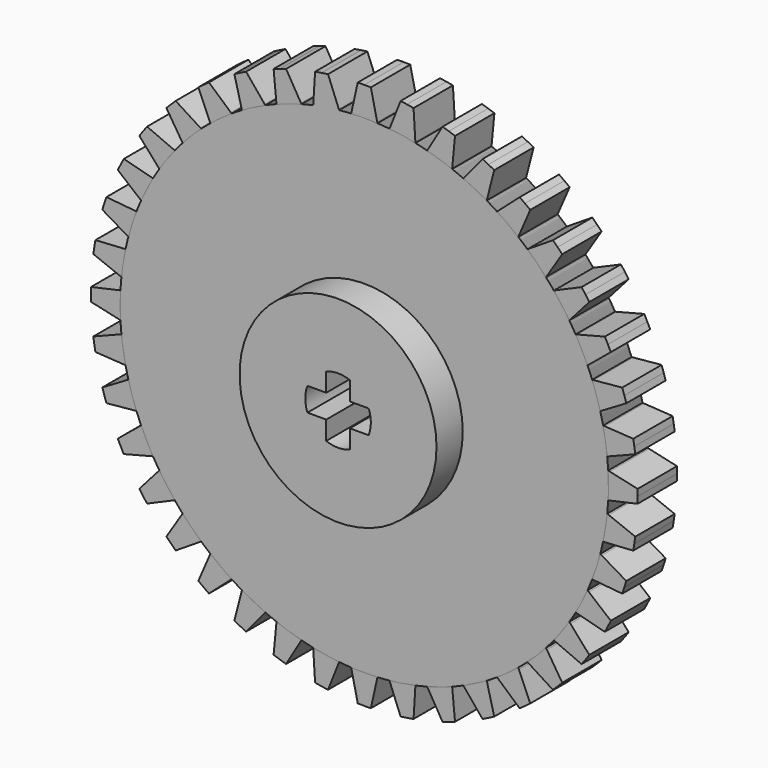
from build123d import *

# Parameters (mm, degrees)
F0_R     = 7.5
F1_DEPTH = 1.875
F3_COUNT = 40
F4_DEPTH = 4.375
F6_DEPTH = 25


with BuildPart() as f1:
    # F0 (on Front) → F1 (new body, symmetric)
    with BuildSketch(Plane.XZ):
        with BuildLine():
            Line((0.7872608089, 3.3734422161), (0.3026279116, 5.5503142364))
            Line((0.3026279116, 5.5503142364), (-0.1973720884, 5.5563175026))
            ThreePointArc((-0.1973720884, 5.5563175026), (-0.4473901074, 5.554816632), (-0.6973720884, 5.5503142364))
            Line((-0.6973720884, 5.5503142364), (-1.1705333394, 3.424970509))
            Line((-1.1705333394, 3.424970509), (-1.1973720884, 3.3044163286))
            ThreePointArc((-1.1973720884, 3.3044163286), (-0.1973720884, 3.3313175026), (0.8026279116, 3.3044163286))
            Line((0.8026279116, 3.3044163286), (0.7872608089, 3.3734422161))
        make_face()
        with BuildLine():
            ThreePointArc((18.4026279116, -15.2686824974), (13.303738977, -2.474934024), (0.8026279116, 3.3044163286))
            ThreePointArc((0.8026279116, 3.3044163286), (-0.1973720884, 3.3313175026), (-1.1973720884, 3.3044163286))
            ThreePointArc((-1.1973720884, 3.3044163286), (-12.9911205618, -28.7697935627), (18.4026279116, -15.2686824974))
        make_face()
        with Locations((-0.1973720884, -15.2686824974)):
            Circle(F0_R, mode=Mode.SUBTRACT)
    extrude(amount=F1_DEPTH, both=True)


with BuildPart() as f3_1:
    # F3: instance of F1
    add(f1.part.rotate(Axis((-0.1973720884, 1.875, -15.2686824974), (0, 1, 0)), 1 * 360 / F3_COUNT))


with BuildPart() as f3_2:
    # F3: instance of F1
    add(f1.part.rotate(Axis((-0.1973720884, 1.875, -15.2686824974), (0, 1, 0)), 2 * 360 / F3_COUNT))


with BuildPart() as f3_3:
    # F3: instance of F1
    add(f1.part.rotate(Axis((-0.1973720884, 1.875, -15.2686824974), (0, 1, 0)), 3 * 360 / F3_COUNT))


with BuildPart() as f3_4:
    # F3: instance of F1
    add(f1.part.rotate(Axis((-0.1973720884, 1.875, -15.2686824974), (0, 1, 0)), 4 * 360 / F3_COUNT))


with BuildPart() as f3_5:
    # F3: instance of F1
    add(f1.part.rotate(Axis((-0.1973720884, 1.875, -15.2686824974), (0, 1, 0)), 5 * 360 / F3_COUNT))


with BuildPart() as f3_6:
    # F3: instance of F1
    add(f1.part.rotate(Axis((-0.1973720884, 1.875, -15.2686824974), (0, 1, 0)), 6 * 360 / F3_COUNT))


with BuildPart() as f3_7:
    # F3: instance of F1
    add(f1.part.rotate(Axis((-0.1973720884, 1.875, -15.2686824974), (0, 1, 0)), 7 * 360 / F3_COUNT))


with BuildPart() as f3_8:
    # F3: instance of F1
    add(f1.part.rotate(Axis((-0.1973720884, 1.875, -15.2686824974), (0, 1, 0)), 8 * 360 / F3_COUNT))


with BuildPart() as f3_9:
    # F3: instance of F1
    add(f1.part.rotate(Axis((-0.1973720884, 1.875, -15.2686824974), (0, 1, 0)), 9 * 360 / F3_COUNT))


with BuildPart() as f3_10:
    # F3: instance of F1
    add(f1.part.rotate(Axis((-0.1973720884, 1.875, -15.2686824974), (0, 1, 0)), 10 * 360 / F3_COUNT))


with BuildPart() as f3_11:
    # F3: instance of F1
    add(f1.part.rotate(Axis((-0.1973720884, 1.875, -15.2686824974), (0, 1, 0)), 11 * 360 / F3_COUNT))


with BuildPart() as f3_12:
    # F3: instance of F1
    add(f1.part.rotate(Axis((-0.1973720884, 1.875, -15.2686824974), (0, 1, 0)), 12 * 360 / F3_COUNT))


with BuildPart() as f3_13:
    # F3: instance of F1
    add(f1.part.rotate(Axis((-0.1973720884, 1.875, -15.2686824974), (0, 1, 0)), 13 * 360 / F3_COUNT))


with BuildPart() as f3_14:
    # F3: instance of F1
    add(f1.part.rotate(Axis((-0.1973720884, 1.875, -15.2686824974), (0, 1, 0)), 14 * 360 / F3_COUNT))


with BuildPart() as f3_15:
    # F3: instance of F1
    add(f1.part.rotate(Axis((-0.1973720884, 1.875, -15.2686824974), (0, 1, 0)), 15 * 360 / F3_COUNT))


with BuildPart() as f3_16:
    # F3: instance of F1
    add(f1.part.rotate(Axis((-0.1973720884, 1.875, -15.2686824974), (0, 1, 0)), 16 * 360 / F3_COUNT))


with BuildPart() as f3_17:
    # F3: instance of F1
    add(f1.part.rotate(Axis((-0.1973720884, 1.875, -15.2686824974), (0, 1, 0)), 17 * 360 / F3_COUNT))


with BuildPart() as f3_18:
    # F3: instance of F1
    add(f1.part.rotate(Axis((-0.1973720884, 1.875, -15.2686824974), (0, 1, 0)), 18 * 360 / F3_COUNT))


with BuildPart() as f3_19:
    # F3: instance of F1
    add(f1.part.rotate(Axis((-0.1973720884, 1.875, -15.2686824974), (0, 1, 0)), 19 * 360 / F3_COUNT))


with BuildPart() as f3_20:
    # F3: instance of F1
    add(f1.part.rotate(Axis((-0.1973720884, 1.875, -15.2686824974), (0, 1, 0)), 20 * 360 / F3_COUNT))


with BuildPart() as f3_21:
    # F3: instance of F1
    add(f1.part.rotate(Axis((-0.1973720884, 1.875, -15.2686824974), (0, 1, 0)), 21 * 360 / F3_COUNT))


with BuildPart() as f3_22:
    # F3: instance of F1
    add(f1.part.rotate(Axis((-0.1973720884, 1.875, -15.2686824974), (0, 1, 0)), 22 * 360 / F3_COUNT))


with BuildPart() as f3_23:
    # F3: instance of F1
    add(f1.part.rotate(Axis((-0.1973720884, 1.875, -15.2686824974), (0, 1, 0)), 23 * 360 / F3_COUNT))


with BuildPart() as f3_24:
    # F3: instance of F1
    add(f1.part.rotate(Axis((-0.1973720884, 1.875, -15.2686824974), (0, 1, 0)), 24 * 360 / F3_COUNT))


with BuildPart() as f3_25:
    # F3: instance of F1
    add(f1.part.rotate(Axis((-0.1973720884, 1.875, -15.2686824974), (0, 1, 0)), 25 * 360 / F3_COUNT))


with BuildPart() as f3_26:
    # F3: instance of F1
    add(f1.part.rotate(Axis((-0.1973720884, 1.875, -15.2686824974), (0, 1, 0)), 26 * 360 / F3_COUNT))


with BuildPart() as f3_27:
    # F3: instance of F1
    add(f1.part.rotate(Axis((-0.1973720884, 1.875, -15.2686824974), (0, 1, 0)), 27 * 360 / F3_COUNT))


with BuildPart() as f3_28:
    # F3: instance of F1
    add(f1.part.rotate(Axis((-0.1973720884, 1.875, -15.2686824974), (0, 1, 0)), 28 * 360 / F3_COUNT))


with BuildPart() as f3_29:
    # F3: instance of F1
    add(f1.part.rotate(Axis((-0.1973720884, 1.875, -15.2686824974), (0, 1, 0)), 29 * 360 / F3_COUNT))


with BuildPart() as f3_30:
    # F3: instance of F1
    add(f1.part.rotate(Axis((-0.1973720884, 1.875, -15.2686824974), (0, 1, 0)), 30 * 360 / F3_COUNT))


with BuildPart() as f3_31:
    # F3: instance of F1
    add(f1.part.rotate(Axis((-0.1973720884, 1.875, -15.2686824974), (0, 1, 0)), 31 * 360 / F3_COUNT))


with BuildPart() as f3_32:
    # F3: instance of F1
    add(f1.part.rotate(Axis((-0.1973720884, 1.875, -15.2686824974), (0, 1, 0)), 32 * 360 / F3_COUNT))


with BuildPart() as f3_33:
    # F3: instance of F1
    add(f1.part.rotate(Axis((-0.1973720884, 1.875, -15.2686824974), (0, 1, 0)), 33 * 360 / F3_COUNT))


with BuildPart() as f3_34:
    # F3: instance of F1
    add(f1.part.rotate(Axis((-0.1973720884, 1.875, -15.2686824974), (0, 1, 0)), 34 * 360 / F3_COUNT))


with BuildPart() as f3_35:
    # F3: instance of F1
    add(f1.part.rotate(Axis((-0.1973720884, 1.875, -15.2686824974), (0, 1, 0)), 35 * 360 / F3_COUNT))


with BuildPart() as f3_36:
    # F3: instance of F1
    add(f1.part.rotate(Axis((-0.1973720884, 1.875, -15.2686824974), (0, 1, 0)), 36 * 360 / F3_COUNT))


with BuildPart() as f3_37:
    # F3: instance of F1
    add(f1.part.rotate(Axis((-0.1973720884, 1.875, -15.2686824974), (0, 1, 0)), 37 * 360 / F3_COUNT))


with BuildPart() as f3_38:
    # F3: instance of F1
    add(f1.part.rotate(Axis((-0.1973720884, 1.875, -15.2686824974), (0, 1, 0)), 38 * 360 / F3_COUNT))


with BuildPart() as f3_39:
    # F3: instance of F1
    add(f1.part.rotate(Axis((-0.1973720884, 1.875, -15.2686824974), (0, 1, 0)), 39 * 360 / F3_COUNT))


with BuildPart() as f4:
    # F0 (on Front) → F4 (new body, symmetric)
    with BuildSketch(Plane.XZ):
        with Locations((-0.1973720884, -15.2686824974)):
            Circle(F0_R)
    extrude(amount=F4_DEPTH, both=True)

    # F5 (on face) → F6 (cut)
    with BuildSketch(Plane.XZ.offset(4.375)):
        with BuildLine():
            ThreePointArc((2.1339367714, -16.1686824974), (2.2593474561, -15.7264270545), (2.3016279116, -15.2686824974))
            ThreePointArc((2.3016279116, -15.2686824974), (2.2593474561, -14.8109379402), (2.1339367714, -14.3686824974))
            Line((2.1339367714, -14.3686824974), (0.7026279116, -14.3686824974))
            Line((0.7026279116, -14.3686824974), (0.7026279116, -12.9373736375))
            ThreePointArc((0.7026279116, -12.9373736375), (-0.1973720884, -12.7696824974), (-1.0973720884, -12.9373736375))
            Line((-1.0973720884, -12.9373736375), (-1.0973720884, -14.3686824974))
            Line((-1.0973720884, -14.3686824974), (-2.5286809483, -14.3686824974))
            ThreePointArc((-2.5286809483, -14.3686824974), (-2.6963720884, -15.2686824974), (-2.5286809483, -16.1686824974))
            Line((-2.5286809483, -16.1686824974), (-1.0973720884, -16.1686824974))
            Line((-1.0973720884, -16.1686824974), (-1.0973720884, -17.5999913572))
            ThreePointArc((-1.0973720884, -17.5999913572), (-0.1973720884, -17.7676824974), (0.7026279116, -17.5999913572))
            Line((0.7026279116, -17.5999913572), (0.7026279116, -16.1686824974))
            Line((0.7026279116, -16.1686824974), (2.1339367714, -16.1686824974))
        make_face()
    extrude(amount=-F6_DEPTH, mode=Mode.SUBTRACT)


solid = Compound([f1.part, f3_1.part, f3_2.part, f3_3.part, f3_4.part, f3_5.part, f3_6.part, f3_7.part, f3_8.part, f3_9.part, f3_10.part, f3_11.part, f3_12.part, f3_13.part, f3_14.part, f3_15.part, f3_16.part, f3_17.part, f3_18.part, f3_19.part, f3_20.part, f3_21.part, f3_22.part, f3_23.part, f3_24.part, f3_25.part, f3_26.part, f3_27.part, f3_28.part, f3_29.part, f3_30.part, f3_31.part, f3_32.part, f3_33.part, f3_34.part, f3_35.part, f3_36.part, f3_37.part, f3_38.part, f3_39.part, f4.part])
